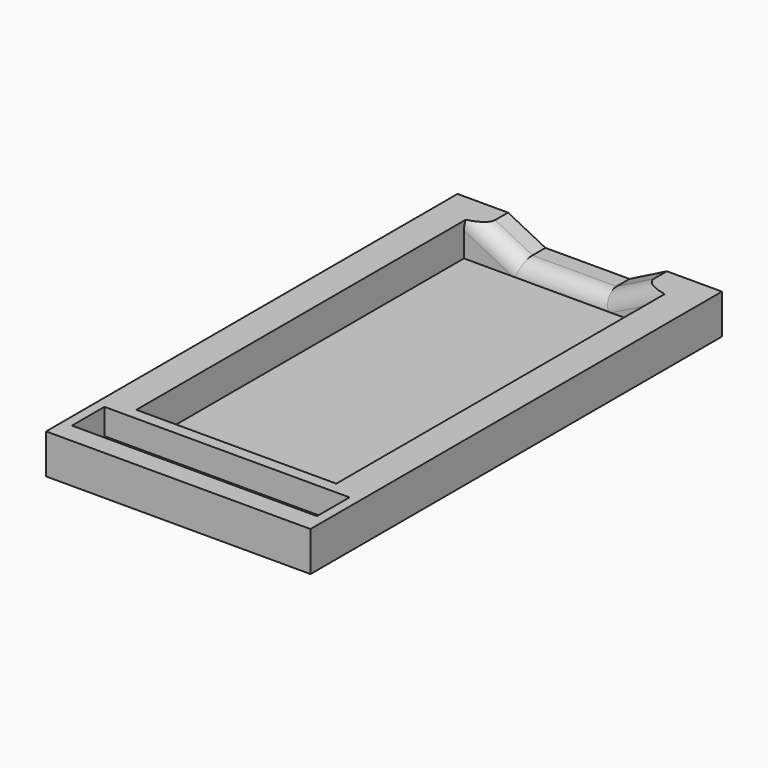
from build123d import *

# Parameters (mm, degrees)
F0_W         = 82
F0_H         = 147
F0_W_2       = 62
F0_H_2       = 127
F1_DEPTH     = 12.3
F2_DEPTH     = 2
F4_DEPTH     = 12.5
F5_W         = 76
F5_H         = 12.6
F6_DEPTH     = 8
F7_DEPTH     = 25
F8_T4_DEPTH  = 38
F8_T10_DEPTH = 50.9116130734
F8_T16_DEPTH = 38
F8_T23_DEPTH = 38
F8_T28_DEPTH = 50.9116130734
F8_T35_DEPTH = 50.9116130734
F8_T39_DEPTH = 38


# Not quite as in the source:
# - a fillet or chamfer that OpenCascade refuses, or shapes differently, is made with other operations: its cross-section is extruded or revolved along the edge and cut away or added


with BuildPart() as f1:
    # F0 (on Top) → F1 (new body)
    with BuildSketch(Plane.XY):
        with Locations((0.9012136459, -11.9470648118)):
            Rectangle(F0_W, F0_H)
        with Locations((0.9012136459, -11.9470648118)):
            Rectangle(F0_W_2, F0_H_2, mode=Mode.SUBTRACT)
    extrude(amount=F1_DEPTH)

    # F0 (on Top) → F2 (join)
    with BuildSketch(Plane.XY):
        with Locations((0.9012136459, -11.9470648118)):
            Rectangle(F0_W_2, F0_H_2)
    extrude(amount=F2_DEPTH)

    # F4 (add): a face of the model
    f4_faces = [f1.faces().sort_by_distance(p)[0] for p in [
        (0.9012136459, -85.4470648118, 6.15),
    ]]
    extrude(f4_faces, amount=F4_DEPTH)

    # F5 (on face) → F6 (cut)
    with BuildSketch(Plane.XY.offset(12.3)):
        with Locations((0.9012136459, -85.3629247222)):
            Rectangle(F5_W, F5_H)
    extrude(amount=-F6_DEPTH, mode=Mode.SUBTRACT)

    # F3 (on face) → F7 (cut)
    with BuildSketch(Plane(origin=(0, 61.5529351882, 0), x_dir=(-1, 0, 0), z_dir=(0, 1, 0))):
        Polygon((24.4224453152, 12.3), (-24.8533971608, 12.3), (-13.251022455, 6.4361359849), (12.8200706095, 6.4361359849), align=None)
    extrude(amount=-F7_DEPTH, mode=Mode.SUBTRACT)

    # F8: fillet of radius 5 on 3 edges, made by hand


with BuildPart() as f8_tool2:
    # F8_s3 → F8_t4 (new body)
    with BuildSketch(Plane(origin=(-1.6465684555, 0, 0.8321790805), x_dir=(0, 1, 0), z_dir=(-0.892490362, 0, 0.4510664627))):
        with BuildLine():
            ThreePointArc((56.5529351882, 0.0385145664), (53.0174012823, 1.5029806605), (51.5529351882, 5.0385145664))
            Line((51.5529351882, 5.0385145664), (51.5529351882, 0.0385145664))
            Line((51.5529351882, 0.0385145664), (56.5529351882, 0.0385145664))
        make_face()
    extrude(amount=F8_T4_DEPTH)

    split(bisect_by=Plane.XY.offset(6.4361359849), keep=Keep.TOP)

    split(bisect_by=Plane.YZ.offset(-30.0987863541), keep=Keep.TOP)


with BuildPart() as f1_1:
    add(f1.part)

    # F8_t1: cut F8_tool2
    add(f8_tool2.part, mode=Mode.SUBTRACT)


with BuildPart() as f8_tool8:
    # F8_s9 → F8_t10 (new body)
    with BuildSketch(Plane.YZ.offset(25.6712824595)):
        with BuildLine():
            ThreePointArc((56.52103919, 6.4361359849), (53.1908229865, 5.1657016483), (51.5529351882, 2))
            Line((51.5529351882, 2), (51.5529351882, 6.4361359849))
            Line((51.5529351882, 6.4361359849), (56.52103919, 6.4361359849))
        make_face()
    extrude(amount=-F8_T10_DEPTH)

    split(bisect_by=Plane(origin=(-0.0173726292, 0, -0.0343738793), x_dir=(0, 1, 0), z_dir=(0.4510664627, 0, 0.892490362)), keep=Keep.TOP)

    split(bisect_by=Plane(origin=(0.1050545028, 0, -0.2078632285), x_dir=(0, 1, 0), z_dir=(-0.4510664627, 0, 0.892490362)), keep=Keep.TOP)


with BuildPart() as f1_2:
    add(f1_1.part)

    # F8_t7: cut F8_tool8
    add(f8_tool8.part, mode=Mode.SUBTRACT)


with BuildPart() as f8_tool14:
    # F8_s15 → F8_t16 (new body)
    with BuildSketch(Plane(origin=(35.9044721827, 0, 18.1461940123), x_dir=(0, 1, 0), z_dir=(-0.892490362, 0, -0.4510664627))):
        with BuildLine():
            ThreePointArc((56.5529351882, 0.232902491), (53.0174012823, 1.6973685851), (51.5529351882, 5.232902491))
            Line((51.5529351882, 5.232902491), (51.5529351882, 0.232902491))
            Line((51.5529351882, 0.232902491), (56.5529351882, 0.232902491))
        make_face()
    extrude(amount=F8_T16_DEPTH)

    split(bisect_by=Plane.XY.offset(6.4361359849), keep=Keep.TOP)

    split(bisect_by=Plane.YZ.offset(31.9012136459), keep=Keep.BOTTOM)


with BuildPart() as f1_3:
    add(f1_2.part)

    # F8_t13: cut F8_tool14
    add(f8_tool14.part, mode=Mode.SUBTRACT)


with BuildPart() as f8_tool21:
    # F8_s22 → F8_t23 (new body)
    with BuildSketch(Plane(origin=(-1.6465684555, 0, 0.8321790805), x_dir=(0, 1, 0), z_dir=(-0.892490362, 0, 0.4510664627))):
        with BuildLine():
            ThreePointArc((56.5529351882, 0.0385145664), (53.0174012823, 1.5029806605), (51.5529351882, 5.0385145664))
            Line((51.5529351882, 5.0385145664), (51.5529351882, 0.0385145664))
            Line((51.5529351882, 0.0385145664), (56.5529351882, 0.0385145664))
        make_face()
    extrude(amount=F8_T23_DEPTH)

    split(bisect_by=Plane.XY.offset(6.4361359849), keep=Keep.BOTTOM)

    split(bisect_by=Plane.XY.offset(2), keep=Keep.TOP)


with BuildPart() as f8_tool26:
    # F8_s27 → F8_t28 (new body)
    with BuildSketch(Plane.YZ.offset(25.6712824595)):
        with BuildLine():
            ThreePointArc((56.52103919, 6.4361359849), (53.1908229865, 5.1657016483), (51.5529351882, 2))
            Line((51.5529351882, 2), (51.5529351882, 6.4361359849))
            Line((51.5529351882, 6.4361359849), (56.52103919, 6.4361359849))
        make_face()
    extrude(amount=-F8_T28_DEPTH)

    split(bisect_by=Plane(origin=(-0.0173726292, 0, -0.0343738793), x_dir=(0, 1, 0), z_dir=(-0.4510664627, 0, -0.892490362)), keep=Keep.TOP)


with BuildPart() as f8_tool21_1:
    add(f8_tool21.part)

    # F8_t30: intersect F8_tool26
    add(f8_tool26.part, mode=Mode.INTERSECT)


with BuildPart() as f1_4:
    add(f1_3.part)

    # F8_t19: cut F8_tool21
    add(f8_tool21_1.part, mode=Mode.SUBTRACT)


with BuildPart() as f8_tool33:
    # F8_s34 → F8_t35 (new body)
    with BuildSketch(Plane.YZ.offset(25.6712824595)):
        with BuildLine():
            ThreePointArc((56.52103919, 6.4361359849), (53.1908229865, 5.1657016483), (51.5529351882, 2))
            Line((51.5529351882, 2), (51.5529351882, 6.4361359849))
            Line((51.5529351882, 6.4361359849), (56.52103919, 6.4361359849))
        make_face()
    extrude(amount=-F8_T35_DEPTH)

    split(bisect_by=Plane(origin=(0.1050545028, 0, -0.2078632285), x_dir=(0, 1, 0), z_dir=(0.4510664627, 0, -0.892490362)), keep=Keep.TOP)


with BuildPart() as f8_tool37:
    # F8_s38 → F8_t39 (new body)
    with BuildSketch(Plane(origin=(35.9044721827, 0, 18.1461940123), x_dir=(0, 1, 0), z_dir=(-0.892490362, 0, -0.4510664627))):
        with BuildLine():
            ThreePointArc((56.5529351882, 0.232902491), (53.0174012823, 1.6973685851), (51.5529351882, 5.232902491))
            Line((51.5529351882, 5.232902491), (51.5529351882, 0.232902491))
            Line((51.5529351882, 0.232902491), (56.5529351882, 0.232902491))
        make_face()
    extrude(amount=F8_T39_DEPTH)

    split(bisect_by=Plane.XY.offset(6.4361359849), keep=Keep.BOTTOM)

    split(bisect_by=Plane.XY.offset(2), keep=Keep.TOP)


with BuildPart() as f8_tool33_1:
    add(f8_tool33.part)

    # F8_t42: intersect F8_tool37
    add(f8_tool37.part, mode=Mode.INTERSECT)


with BuildPart() as f1_5:
    add(f1_4.part)

    # F8_t31: cut F8_tool33
    add(f8_tool33_1.part, mode=Mode.SUBTRACT)


solid = f1_5.part
